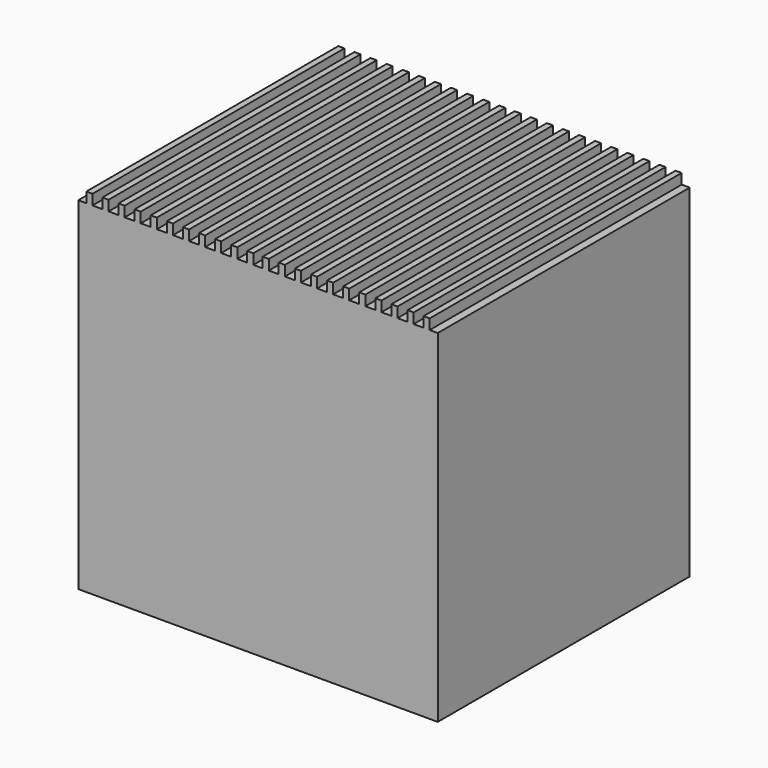
from build123d import *

# Parameters (mm, degrees)
F2_W         = 10.5
F2_H         = 9.2
F3_DEPTH     = 10
F4_W         = 0.18
F4_H         = 9.2
F5_DEPTH     = 0.3
F6_DEPTH     = 0.3
F7_TEXT_SIZE = 6.5381177372
F8_DEPTH     = 2


# Not quite as in the source:
# - Text() gives the source's letters only with a copy of the font that has no kerning and outlines rounded to 1/6400 em; it was checked with that copy


with BuildPart() as f3:
    # F2 (on Top) → F3 (new body)
    with BuildSketch(Plane.XY):
        Rectangle(F2_W, F2_H)
    extrude(amount=F3_DEPTH)

    # F4 (on face) → F5 (join)
    with BuildSketch(Plane.XY.offset(10)):
        with Locations((0.225, 0)):
            Rectangle(F4_W, F4_H)
        with Locations((0.695, 0)):
            Rectangle(F4_W, F4_H)
        with Locations((-0.225, 0)):
            Rectangle(F4_W, F4_H)
        with Locations((1.165, 0)):
            Rectangle(F4_W, F4_H)
        with Locations((1.635, 0)):
            Rectangle(F4_W, F4_H)
        with Locations((2.105, 0)):
            Rectangle(F4_W, F4_H)
        with Locations((2.575, 0)):
            Rectangle(F4_W, F4_H)
        with Locations((3.045, 0)):
            Rectangle(F4_W, F4_H)
        with Locations((3.515, 0)):
            Rectangle(F4_W, F4_H)
        with Locations((3.985, 0)):
            Rectangle(F4_W, F4_H)
        with Locations((4.455, 0)):
            Rectangle(F4_W, F4_H)
        with Locations((4.925, 0)):
            Rectangle(F4_W, F4_H)
        with Locations((-4.455, 0)):
            Rectangle(F4_W, F4_H)
        with Locations((-4.925, 0)):
            Rectangle(F4_W, F4_H)
        with Locations((-3.045, 0)):
            Rectangle(F4_W, F4_H)
        with Locations((-2.105, 0)):
            Rectangle(F4_W, F4_H)
        with Locations((-2.575, 0)):
            Rectangle(F4_W, F4_H)
        with Locations((-1.165, 0)):
            Rectangle(F4_W, F4_H)
        with Locations((-3.985, 0)):
            Rectangle(F4_W, F4_H)
        with Locations((-0.695, 0)):
            Rectangle(F4_W, F4_H)
        with Locations((-3.515, 0)):
            Rectangle(F4_W, F4_H)
        with Locations((-1.635, 0)):
            Rectangle(F4_W, F4_H)
    extrude(amount=F5_DEPTH)

    # F4 (on face) → F6 (join)
    with BuildSketch(Plane.XY.offset(10)):
        with Locations((0.225, 0)):
            Rectangle(F4_W, F4_H)
        with Locations((0.695, 0)):
            Rectangle(F4_W, F4_H)
        with Locations((-0.225, 0)):
            Rectangle(F4_W, F4_H)
        with Locations((1.165, 0)):
            Rectangle(F4_W, F4_H)
        with Locations((1.635, 0)):
            Rectangle(F4_W, F4_H)
        with Locations((2.105, 0)):
            Rectangle(F4_W, F4_H)
        with Locations((2.575, 0)):
            Rectangle(F4_W, F4_H)
        with Locations((3.045, 0)):
            Rectangle(F4_W, F4_H)
        with Locations((3.515, 0)):
            Rectangle(F4_W, F4_H)
        with Locations((3.985, 0)):
            Rectangle(F4_W, F4_H)
        with Locations((4.455, 0)):
            Rectangle(F4_W, F4_H)
        with Locations((4.925, 0)):
            Rectangle(F4_W, F4_H)
        with Locations((-4.455, 0)):
            Rectangle(F4_W, F4_H)
        with Locations((-4.925, 0)):
            Rectangle(F4_W, F4_H)
        with Locations((-3.045, 0)):
            Rectangle(F4_W, F4_H)
        with Locations((-2.105, 0)):
            Rectangle(F4_W, F4_H)
        with Locations((-2.575, 0)):
            Rectangle(F4_W, F4_H)
        with Locations((-1.165, 0)):
            Rectangle(F4_W, F4_H)
        with Locations((-3.985, 0)):
            Rectangle(F4_W, F4_H)
        with Locations((-0.695, 0)):
            Rectangle(F4_W, F4_H)
        with Locations((-3.515, 0)):
            Rectangle(F4_W, F4_H)
        with Locations((-1.635, 0)):
            Rectangle(F4_W, F4_H)
    extrude(amount=F6_DEPTH)

    # F7 (on face) → F8 (cut)
    with BuildSketch(Plane(origin=(0, 0, 0), x_dir=(1, 0, 0), z_dir=(0, 0, -1))):
        with Locations((-3.9913304852, -2.3895113771)):
            Text('2b', F7_TEXT_SIZE, font='Open Sans', font_style=FontStyle.BOLD, text_align=(TextAlign.LEFT, TextAlign.BOTTOM))
    extrude(amount=-F8_DEPTH, mode=Mode.SUBTRACT)


solid = f3.part
